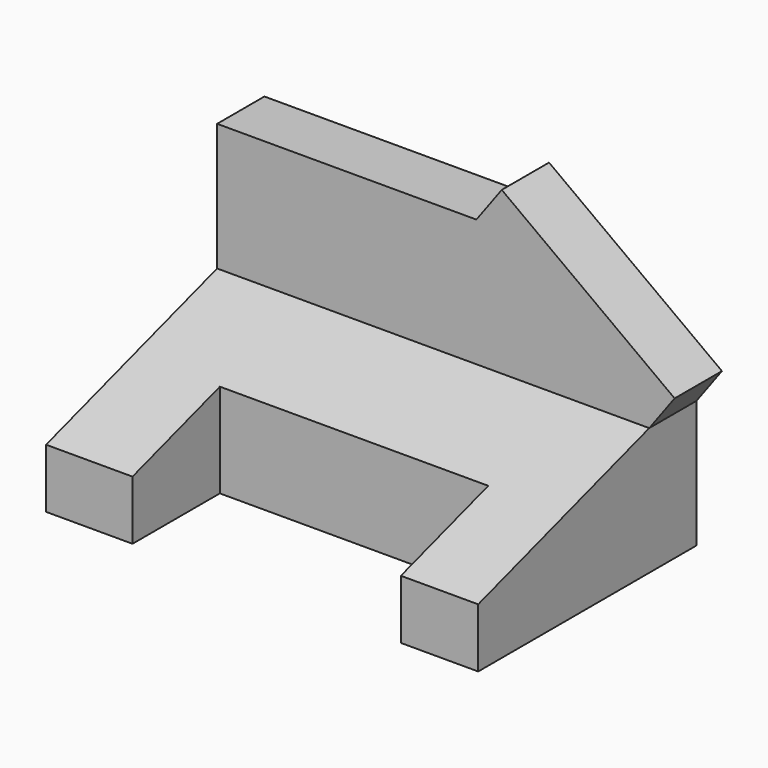
from build123d import *

# Parameters (mm, degrees)
F1_DEPTH = 95
F3_DEPTH = 13.001
F4_W     = 59
F4_H     = 24
F5_DEPTH = 56.001
F6_DEPTH = 9.4


# Not quite as in the source:
# - a feature names something its author has since deleted; it is built from what else it names


with BuildPart() as f1:
    # F0 (on Right) → F1 (new body)
    with BuildSketch(Plane.YZ):
        Polygon((-60, 13), (-60, 0), (0, 0), (0, 56), (-13, 56), (-13, 28), align=None)
    extrude(amount=F1_DEPTH)

    # F2 (on face) → F3 (cut, through all)
    with BuildSketch(Plane.XZ.offset(13)):
        Polygon((95, 56), (57, 56), (95, 28), align=None)
    extrude(amount=-F3_DEPTH, mode=Mode.SUBTRACT)

    # F4 (on face) → F5 (cut, through all)
    with BuildSketch(Plane(origin=(0, 0, 0), x_dir=(1, 0, 0), z_dir=(0, 0, -1))):
        with Locations((48.5, 48)):
            Rectangle(F4_W, F4_H)
    extrude(amount=-F5_DEPTH, mode=Mode.SUBTRACT)

    # F6 (add): a face of the model
    f6_faces = [f1.faces().sort_by_distance(p)[0] for p in [
        (76, -6.5, 42),
    ]]
    extrude(f6_faces, amount=F6_DEPTH)


solid = f1.part
